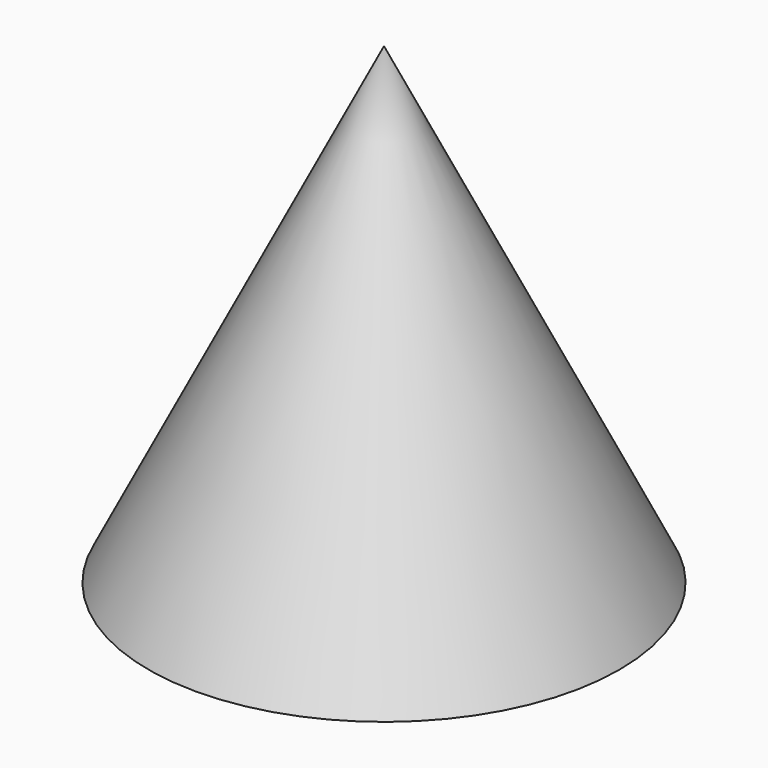
from build123d import *

# Parameters (mm, degrees)
F0_R     = 25
F1_DEPTH = 50


# Not quite as in the source:
# - a fillet or chamfer that OpenCascade refuses, or shapes differently, is made with other operations: its cross-section is extruded or revolved along the edge and cut away or added


with BuildPart() as f1:
    # F0 (on Top) → F1 (new body)
    with BuildSketch(Plane.XY):
        Circle(F0_R)
    extrude(amount=F1_DEPTH)

    # F2: chamfer of 25 x 50.1422427065 on 1 edges, made by hand

    # F2_s1 → F2_t2 (revolve, cut)
    with BuildSketch(Plane.XZ):
        Polygon((25, -0.1422427065), (0, 50), (25, 50), align=None)
    revolve(axis=Axis((0, 0, 50), (0, 0, 1)), mode=Mode.SUBTRACT)


solid = f1.part
